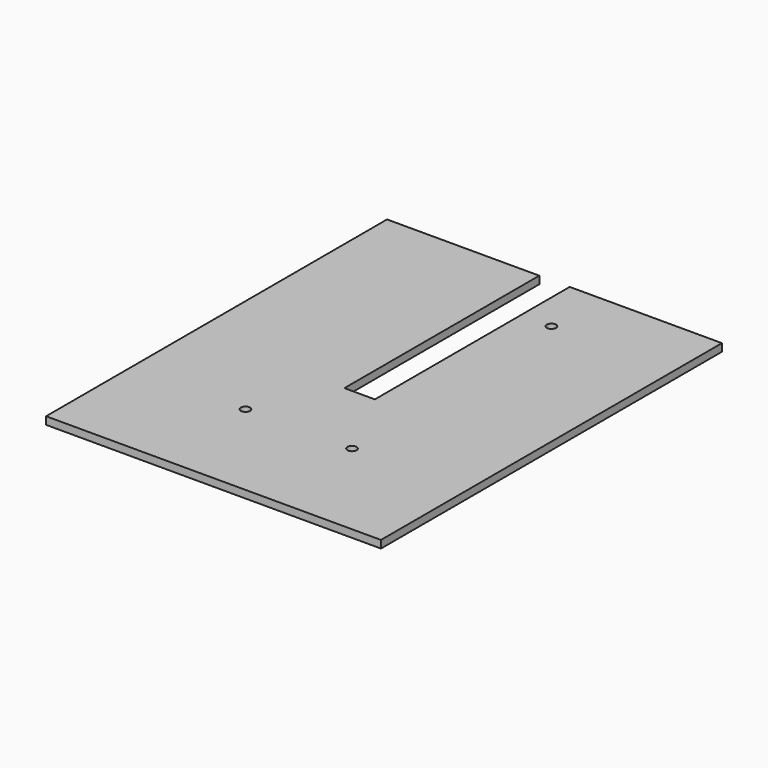
from build123d import *

# Parameters (mm, degrees)
F0_R     = 1.905
F1_DEPTH = 3.175


# Not quite as in the source:
# - a length typed as a fraction of an inch, garbled in the dataset ("3 / 203.2 mm" for 3/8 in), is restored


with BuildPart() as f1:
    # F0 (on Top) → F1 (new body)
    with BuildSketch(Plane.XY):
        Polygon((63.5, 177.8), (0, 177.8), (0, 0), (139.7, 0), (139.7, 177.8), (76.2, 177.8), (76.2, 76.2), (63.5, 76.2), align=None)
        with Locations((47.625, 44.45)):
            Circle(F0_R, mode=Mode.SUBTRACT)
        with Locations((92.075, 44.45)):
            Circle(F0_R, mode=Mode.SUBTRACT)
        with Locations((88.9, 152.4)):
            Circle(F0_R, mode=Mode.SUBTRACT)
    extrude(amount=F1_DEPTH)


solid = f1.part
